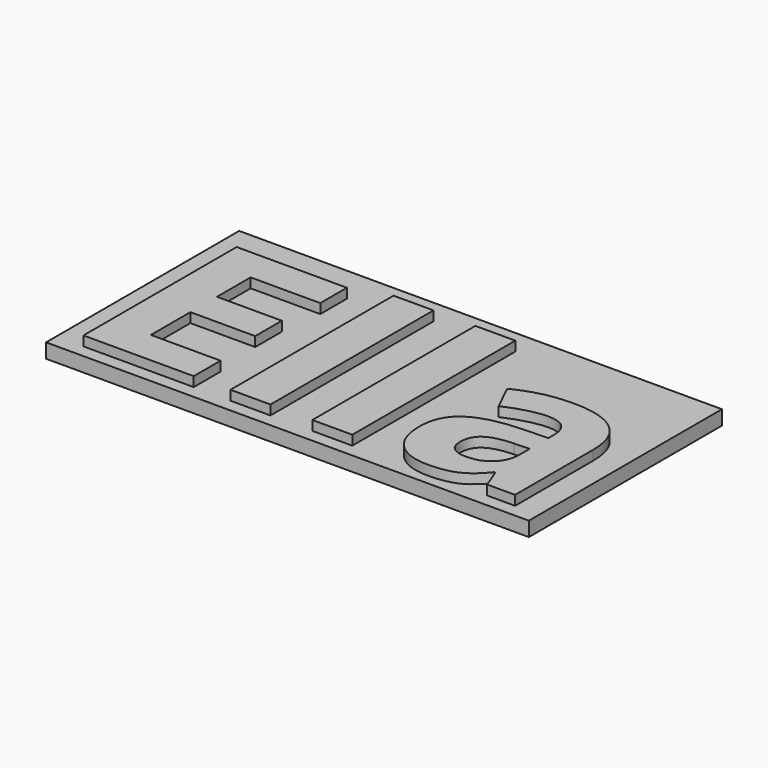
from build123d import *

# Parameters (mm, degrees)
F0_W         = 100
F0_H         = 50
F1_DEPTH     = 3
F2_TEXT_SIZE = 55.5555555556
F3_DEPTH     = 2


# Not quite as in the source:
# - Text() gives the source's letters only with a copy of the font that has no kerning and outlines rounded to 1/6400 em; it was checked with that copy


with BuildPart() as f1:
    # F0 (on Top) → F1 (new body)
    with BuildSketch(Plane.XY):
        with Locations((-50, 25)):
            Rectangle(F0_W, F0_H)
    extrude(amount=F1_DEPTH)

    # F2 (on face) → F3 (join)
    with BuildSketch(Plane.XY.offset(3)):
        with Locations((-99.3822556169, 2.6701185499)):
            Text('Ella', F2_TEXT_SIZE, font='Open Sans', font_style=FontStyle.BOLD, text_align=(TextAlign.LEFT, TextAlign.BOTTOM))
    extrude(amount=F3_DEPTH)


solid = f1.part
